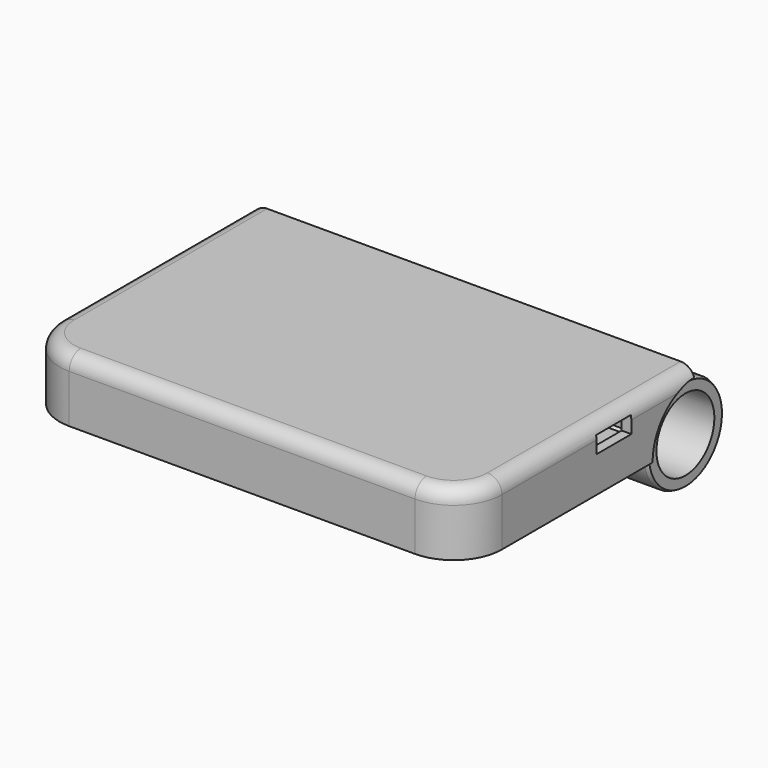
from build123d import *
from build123d import SkipClean  # not in build123d's __all__

# Parameters (mm, degrees)
F0_W           = 116.3828
F0_H           = 76.2
F1_DEPTH       = 16.51
F2_R           = 12.7
F3_DEPTH       = 58.1914
F4_R           = 12.7
F6_DEPTH       = 15.875
F7_R           = 6.985
F10_DEPTH      = 53.34
F10_DEPTH_BACK = 53.34
F11_W          = 19.05
F11_H          = 5.715
F12_DEPTH      = 17.78
F13_W          = 20.32
F13_H          = 11.43
F14_DEPTH      = 1.27
F16_DEPTH      = 25.4
F17_R          = 5.08
F18_W          = 7.9625188272
F18_H          = 24.355364847
F18_W_2        = 74.197281152
F18_H_2        = 2.5465525687
F19_DEPTH      = 5.08
F20_T1_DEPTH   = 73.025
F20_T3_DEPTH   = 90.9828
F20_T6_ANGLE   = 90
F20_T8_ANGLE   = 90
F21_R          = 5.08
F22_R          = 13.97
F23_DEPTH      = 2.54
F24_R          = 13.97
F25_DEPTH      = 2.54
F26_R          = 9.525
F27_DEPTH      = 63.5
F29_DEPTH      = 25.4
F31_DEPTH      = 63.5


# Not quite as in the source:
# - a fillet or chamfer that OpenCascade refuses, or shapes differently, is made with other operations: its cross-section is extruded or revolved along the edge and cut away or added


with BuildPart() as f1:
    # F0 (on Top) → F1 (new body)
    with BuildSketch(Plane.XY):
        Rectangle(F0_W, F0_H)
    extrude(amount=F1_DEPTH)

    # F2 (on Right) → F3 (join, symmetric)
    with BuildSketch(Plane.YZ):
        with Locations((38.1, 0)):
            Circle(F2_R)
    extrude(amount=F3_DEPTH, both=True)

    # F4
    f4_edges = [f1.edges().sort_by_distance(p)[0] for p in [
        (-58.1914, -38.1, 8.255),
        (58.1914, -38.1, 8.255),
    ]]
    fillet(f4_edges, radius=F4_R)

    # F5 (on face) → F6 (cut)
    with BuildSketch(Plane(origin=(0, 0, 0), x_dir=(1, 0, 0), z_dir=(0, 0, -1))):
        with BuildLine():
            Line((-54.3814, 25.4), (-54.3814, -21.59))
            Line((-54.3814, -21.59), (54.3814, -21.59))
            Line((54.3814, -21.59), (54.3814, 25.4))
            ThreePointArc((54.3814, 25.4), (51.7775792847, 31.6861792847), (45.4914, 34.29))
            Line((45.4914, 34.29), (-45.4914, 34.29))
            ThreePointArc((-45.4914, 34.29), (-51.7775792847, 31.6861792847), (-54.3814, 25.4))
        make_face()
    extrude(amount=-F6_DEPTH, mode=Mode.SUBTRACT)

    # F8 (on Top) → F9 (revolve, cut)
    with BuildSketch(Plane.XY):
        Polygon((-30.48, 28.575), (-30.48, 25.4), (-30.48, 24.13), (30.48, 24.13), (30.48, 25.4), (30.48, 28.575), (24.13, 28.575), (19.05, 28.575), (19.05, 38.1), (0, 38.1), (-19.05, 38.1), (-19.05, 28.575), (-24.13, 28.575), align=None)
    revolve(axis=Axis((-9.525, 38.1, 0), (1, 0, 0)), mode=Mode.SUBTRACT)

    # F7 (on Right) → F10 (cut, two sides)
    with BuildSketch(Plane.YZ) as f10_sk:
        with Locations((38.1, 0)):
            Circle(F7_R)
    extrude(amount=F10_DEPTH, mode=Mode.SUBTRACT)
    extrude(f10_sk.sketch, amount=-F10_DEPTH_BACK, mode=Mode.SUBTRACT)

    # F11 (on face) → F12 (cut)
    with BuildSketch(Plane.XZ.offset(-21.59)):
        with Locations((44.8564, 4.1275)):
            Rectangle(F11_W, F11_H)
        with Locations((-44.8564, 4.1275)):
            Rectangle(F11_W, F11_H)
    extrude(amount=-F12_DEPTH, mode=Mode.SUBTRACT)

    # F13 (on face) → F14 (cut)
    with BuildSketch(Plane(origin=(54.3814, 0, 0), x_dir=(0, -1, 0), z_dir=(-1, 0, 0))):
        with Locations((-11.43, 10.16)):
            Rectangle(F13_W, F13_H)
    extrude(amount=-F14_DEPTH, mode=Mode.SUBTRACT)

    # F15 (on face) → F16 (cut)
    with BuildSketch(Plane(origin=(55.6514, 0, 0), x_dir=(0, -1, 0), z_dir=(-1, 0, 0))):
        Polygon((-17.145, 9.4234), (-5.715, 9.4234), (-5.715, 13.7922), (-11.43, 13.7922), (-17.145, 13.7922), align=None)
    extrude(amount=-F16_DEPTH, mode=Mode.SUBTRACT)

    # F17
    f17_edges = [f1.edges().sort_by_distance(p)[0] for p in [
        (-54.3814, -1.905, 15.875),
    ]]
    fillet(f17_edges, radius=F17_R)

    # F18 (on face) → F19 (join)
    with BuildSketch(Plane(origin=(0, 0, 15.875), x_dir=(1, 0, 0), z_dir=(0, 0, -1))):
        with Locations((52.2920594136, 10.7005844475)):
            Rectangle(F18_W, F18_H)
        Polygon((-35.9664, -19.1008), (-35.9664, -8.3696618676), (-39.6496931181, -8.3696618676), (-39.6496931181, -22.3802613997), (-21.43734819, -22.3802613997), (-21.43734819, -19.1008), align=None)
        with Locations((5.3238477558, 34.0265762843)):
            Rectangle(F18_W_2, F18_H_2)
    extrude(amount=F19_DEPTH)

    # F20: fillet of radius 3.81 on 1 edges, made by hand

    # F20_s2 → F20_t1 (cut)
    with BuildSketch(Plane.XZ.offset(-47.625)):
        with BuildLine():
            ThreePointArc((-58.1914, 12.7), (-57.0754768363, 15.3940768363), (-54.3814, 16.51))
            Line((-54.3814, 16.51), (-58.1914, 16.51))
            Line((-58.1914, 16.51), (-58.1914, 12.7))
        make_face()
        with BuildLine():
            ThreePointArc((58.1914, 12.7), (57.0754768363, 15.3940768363), (54.3814, 16.51))
            Line((54.3814, 16.51), (58.1914, 16.51))
            Line((58.1914, 16.51), (58.1914, 12.7))
        make_face()
    extrude(amount=F20_T1_DEPTH, mode=Mode.SUBTRACT)

    # F20_s4 → F20_t3 (cut)
    with BuildSketch(Plane.YZ.offset(-45.4914)):
        with BuildLine():
            ThreePointArc((-38.1, 12.7), (-36.9840768363, 15.3940768363), (-34.29, 16.51))
            Line((-34.29, 16.51), (-38.1, 16.51))
            Line((-38.1, 16.51), (-38.1, 12.7))
        make_face()
    extrude(amount=F20_T3_DEPTH, mode=Mode.SUBTRACT)

    # F20_s5 → F20_t6 (revolve, cut)
    with BuildSketch(Plane.XZ.offset(25.4)):
        with BuildLine():
            ThreePointArc((-58.1914, 12.7), (-57.0754768363, 15.3940768363), (-54.3814, 16.51))
            Line((-54.3814, 16.51), (-58.1914, 16.51))
            Line((-58.1914, 16.51), (-58.1914, 12.7))
        make_face()
    revolve(axis=Axis((-45.4914, -25.4, 16.51), (0, 0, 1)), revolution_arc=F20_T6_ANGLE, mode=Mode.SUBTRACT)

    # F20_s7 → F20_t8 (revolve, cut)
    with BuildSketch(Plane.XZ.offset(25.4)):
        with BuildLine():
            ThreePointArc((58.1914, 12.7), (57.0754768363, 15.3940768363), (54.3814, 16.51))
            Line((54.3814, 16.51), (58.1914, 16.51))
            Line((58.1914, 16.51), (58.1914, 12.7))
        make_face()
    revolve(axis=Axis((45.4914, -25.4, 16.51), (0, 0, -1)), revolution_arc=F20_T8_ANGLE, mode=Mode.SUBTRACT)

    # F21
    f21_edges = [f1.edges().sort_by_distance(p)[0] for p in [
        (58.1914, 47.080256, -8.980256),
        (-58.1914, 47.080256, -8.980256),
    ]]
    fillet(f21_edges, radius=F21_R)

    # F22 (on face) → F23 (cut)
    with BuildSketch(Plane(origin=(-58.1914, 0, 0), x_dir=(0, -1, 0), z_dir=(-1, 0, 0))):
        with Locations((-38.1, 0)):
            Circle(F22_R)
    extrude(amount=-F23_DEPTH, mode=Mode.SUBTRACT)

    # F24 (on face) → F25 (cut)
    with BuildSketch(Plane.YZ.offset(58.1914)):
        with Locations((38.1, 0)):
            Circle(F24_R)
    extrude(amount=-F25_DEPTH, mode=Mode.SUBTRACT)

    # F26 (on Right) → F27 (cut, symmetric)
    with BuildSketch(Plane.YZ):
        with Locations((38.1, 0)):
            Circle(F26_R)
    extrude(amount=F27_DEPTH, both=True, mode=Mode.SUBTRACT)

    # F28 (on face) → F29 (cut)
    with BuildSketch(Plane.XZ.offset(-21.59)):
        with BuildLine():
            ThreePointArc((12.065, 9.6555790053), (10.5771024484, 13.2476814537), (6.985, 14.7355790053))
            Line((6.985, 14.7355790053), (-6.985, 14.7355790053))
            ThreePointArc((-6.985, 14.7355790053), (-10.5771024484, 13.2476814537), (-12.065, 9.6555790053))
            Line((-12.065, 9.6555790053), (-12.065, 8.4972062227))
            ThreePointArc((-12.065, 8.4972062227), (-10.5771024484, 4.9051037742), (-6.985, 3.4172062227))
            Line((-6.985, 3.4172062227), (6.985, 3.4172062227))
            ThreePointArc((6.985, 3.4172062227), (10.5771024484, 4.9051037742), (12.065, 8.4972062227))
            Line((12.065, 8.4972062227), (12.065, 9.6555790053))
        make_face()
    extrude(amount=-F29_DEPTH, mode=Mode.SUBTRACT)

    # F30 (on Right) → F31 (cut, symmetric)
    with BuildSketch(Plane.YZ):
        with BuildLine():
            ThreePointArc((38.1, 12.446), (46.9006509986, -8.8006509986), (25.654, 0))
            Line((25.654, 0), (20.574, 0))
            Line((20.574, 0), (20.574, -20.574))
            Line((20.574, -20.574), (58.674, -20.574))
            Line((58.674, -20.574), (58.674, 17.526))
            Line((58.674, 17.526), (38.1, 17.526))
            Line((38.1, 17.526), (38.1, 12.446))
        make_face()
    with SkipClean():  # cleaning this boolean's faces spoils the solid; the shape is the same uncleaned
        extrude(amount=F31_DEPTH, both=True, mode=Mode.SUBTRACT)


solid = f1.part
